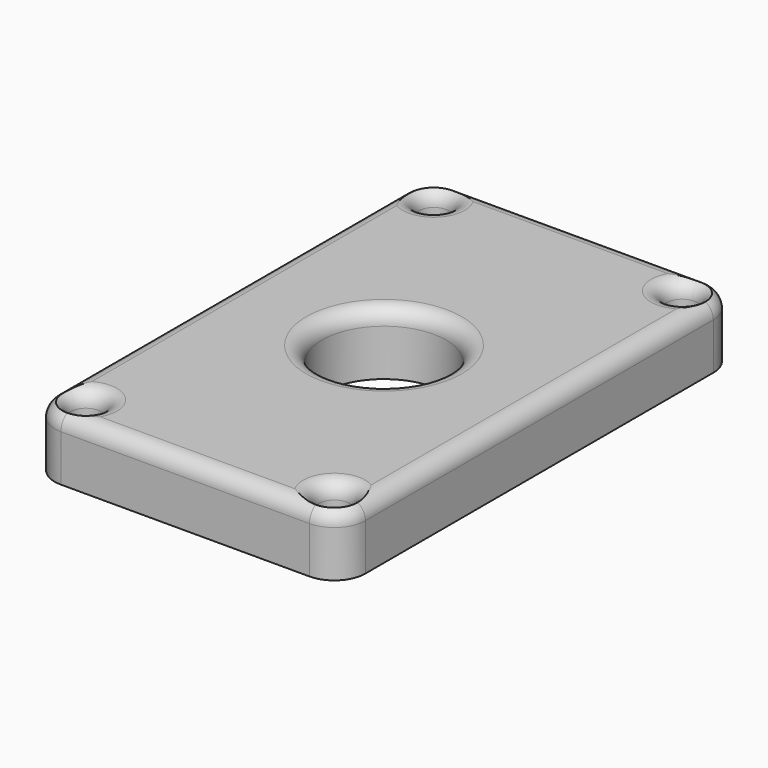
from build123d import *

# Parameters (mm, degrees)
F0_R         = 3.175
F0_R_2       = 12.7
F1_DEPTH     = 12.7
F2_T1_DEPTH  = 50.8
F2_T3_DEPTH  = 88.9
F2_T6_ANGLE  = 90
F2_T8_ANGLE  = 90
F2_T10_ANGLE = 90
F2_T12_ANGLE = 90


# Not quite as in the source:
# - a fillet or chamfer that OpenCascade refuses, or shapes differently, is made with other operations: its cross-section is extruded or revolved along the edge and cut away or added


with BuildPart() as f1:
    # F0 (on Top) → F1 (new body)
    with BuildSketch(Plane.XY):
        with BuildLine():
            ThreePointArc((31.75, 44.45), (29.8901280605, 48.9401280605), (25.4, 50.8))
            Line((25.4, 50.8), (-25.4, 50.8))
            ThreePointArc((-25.4, 50.8), (-29.8901280605, 48.9401280605), (-31.75, 44.45))
            Line((-31.75, 44.45), (-31.75, -44.45))
            ThreePointArc((-31.75, -44.45), (-29.8901280605, -48.9401280605), (-25.4, -50.8))
            Line((-25.4, -50.8), (25.4, -50.8))
            ThreePointArc((25.4, -50.8), (29.8901280605, -48.9401280605), (31.75, -44.45))
            Line((31.75, -44.45), (31.75, 44.45))
        make_face()
        with Locations((-25.4, -44.45)):
            Circle(F0_R, mode=Mode.SUBTRACT)
        with Locations((25.4, -44.45)):
            Circle(F0_R, mode=Mode.SUBTRACT)
        Circle(F0_R_2, mode=Mode.SUBTRACT)
        with Locations((-25.4, 44.45)):
            Circle(F0_R, mode=Mode.SUBTRACT)
        with Locations((25.4, 44.45)):
            Circle(F0_R, mode=Mode.SUBTRACT)
    extrude(amount=F1_DEPTH)

    # F2: fillet of radius 3.175 on 13 edges, made by hand

    # F2_s2 → F2_t1 (cut)
    with BuildSketch(Plane.YZ.offset(-25.4)):
        with BuildLine():
            ThreePointArc((50.8, 9.525), (49.8700640303, 11.7700640303), (47.625, 12.7))
            Line((47.625, 12.7), (50.8, 12.7))
            Line((50.8, 12.7), (50.8, 9.525))
        make_face()
        with BuildLine():
            ThreePointArc((-50.8, 9.525), (-49.8700640303, 11.7700640303), (-47.625, 12.7))
            Line((-47.625, 12.7), (-50.8, 12.7))
            Line((-50.8, 12.7), (-50.8, 9.525))
        make_face()
    extrude(amount=F2_T1_DEPTH, mode=Mode.SUBTRACT)

    # F2_s4 → F2_t3 (cut)
    with BuildSketch(Plane.XZ.offset(-44.45)):
        with BuildLine():
            ThreePointArc((-31.75, 9.525), (-30.8200640303, 11.7700640303), (-28.575, 12.7))
            Line((-28.575, 12.7), (-31.75, 12.7))
            Line((-31.75, 12.7), (-31.75, 9.525))
        make_face()
        with BuildLine():
            ThreePointArc((31.75, 9.525), (30.8200640303, 11.7700640303), (28.575, 12.7))
            Line((28.575, 12.7), (31.75, 12.7))
            Line((31.75, 12.7), (31.75, 9.525))
        make_face()
    extrude(amount=F2_T3_DEPTH, mode=Mode.SUBTRACT)

    # F2_s5 → F2_t6 (revolve, cut)
    with BuildSketch(Plane.XZ.offset(-44.45)):
        with BuildLine():
            ThreePointArc((31.75, 9.525), (30.8200640303, 11.7700640303), (28.575, 12.7))
            Line((28.575, 12.7), (31.75, 12.7))
            Line((31.75, 12.7), (31.75, 9.525))
        make_face()
    revolve(axis=Axis((25.4, 44.45, 12.7), (0, 0, 1)), revolution_arc=F2_T6_ANGLE, mode=Mode.SUBTRACT)

    # F2_s7 → F2_t8 (revolve, cut)
    with BuildSketch(Plane.YZ.offset(-25.4)):
        with BuildLine():
            ThreePointArc((50.8, 9.525), (49.8700640303, 11.7700640303), (47.625, 12.7))
            Line((47.625, 12.7), (50.8, 12.7))
            Line((50.8, 12.7), (50.8, 9.525))
        make_face()
    revolve(axis=Axis((-25.4, 44.45, 12.7), (0, 0, 1)), revolution_arc=F2_T8_ANGLE, mode=Mode.SUBTRACT)

    # F2_s9 → F2_t10 (revolve, cut)
    with BuildSketch(Plane.XZ.offset(44.45)):
        with BuildLine():
            ThreePointArc((-31.75, 9.525), (-30.8200640303, 11.7700640303), (-28.575, 12.7))
            Line((-28.575, 12.7), (-31.75, 12.7))
            Line((-31.75, 12.7), (-31.75, 9.525))
        make_face()
    revolve(axis=Axis((-25.4, -44.45, 12.7), (0, 0, 1)), revolution_arc=F2_T10_ANGLE, mode=Mode.SUBTRACT)

    # F2_s11 → F2_t12 (revolve, cut)
    with BuildSketch(Plane.YZ.offset(25.4)):
        with BuildLine():
            ThreePointArc((-50.8, 9.525), (-49.8700640303, 11.7700640303), (-47.625, 12.7))
            Line((-47.625, 12.7), (-50.8, 12.7))
            Line((-50.8, 12.7), (-50.8, 9.525))
        make_face()
    revolve(axis=Axis((25.4, -44.45, 12.7), (0, 0, 1)), revolution_arc=F2_T12_ANGLE, mode=Mode.SUBTRACT)

    # F2_s13 → F2_t14 (revolve, cut)
    with BuildSketch(Plane.XZ.offset(44.45)):
        with BuildLine():
            ThreePointArc((-22.225, 9.525), (-21.2950640303, 11.7700640303), (-19.05, 12.7))
            Line((-19.05, 12.7), (-22.225, 12.7))
            Line((-22.225, 12.7), (-22.225, 9.525))
        make_face()
    revolve(axis=Axis((-25.4, -44.45, 12.7), (0, 0, 1)), mode=Mode.SUBTRACT)

    # F2_s15 → F2_t16 (revolve, cut)
    with BuildSketch(Plane.XZ.offset(44.45)):
        with BuildLine():
            ThreePointArc((28.575, 9.525), (29.5049359697, 11.7700640303), (31.75, 12.7))
            Line((31.75, 12.7), (28.575, 12.7))
            Line((28.575, 12.7), (28.575, 9.525))
        make_face()
    revolve(axis=Axis((25.4, -44.45, 12.7), (0, 0, 1)), mode=Mode.SUBTRACT)

    # F2_s17 → F2_t18 (revolve, cut)
    with BuildSketch(Plane.XZ):
        with BuildLine():
            ThreePointArc((12.7, 9.525), (13.6299359697, 11.7700640303), (15.875, 12.7))
            Line((15.875, 12.7), (12.7, 12.7))
            Line((12.7, 12.7), (12.7, 9.525))
        make_face()
    revolve(axis=Axis((0, 0, 12.7), (0, 0, 1)), mode=Mode.SUBTRACT)

    # F2_s19 → F2_t20 (revolve, cut)
    with BuildSketch(Plane.XZ.offset(-44.45)):
        with BuildLine():
            ThreePointArc((-22.225, 9.525), (-21.2950640303, 11.7700640303), (-19.05, 12.7))
            Line((-19.05, 12.7), (-22.225, 12.7))
            Line((-22.225, 12.7), (-22.225, 9.525))
        make_face()
    revolve(axis=Axis((-25.4, 44.45, 12.7), (0, 0, 1)), mode=Mode.SUBTRACT)

    # F2_s21 → F2_t22 (revolve, cut)
    with BuildSketch(Plane.XZ.offset(-44.45)):
        with BuildLine():
            ThreePointArc((28.575, 9.525), (29.5049359697, 11.7700640303), (31.75, 12.7))
            Line((31.75, 12.7), (28.575, 12.7))
            Line((28.575, 12.7), (28.575, 9.525))
        make_face()
    revolve(axis=Axis((25.4, 44.45, 12.7), (0, 0, 1)), mode=Mode.SUBTRACT)


solid = f1.part
